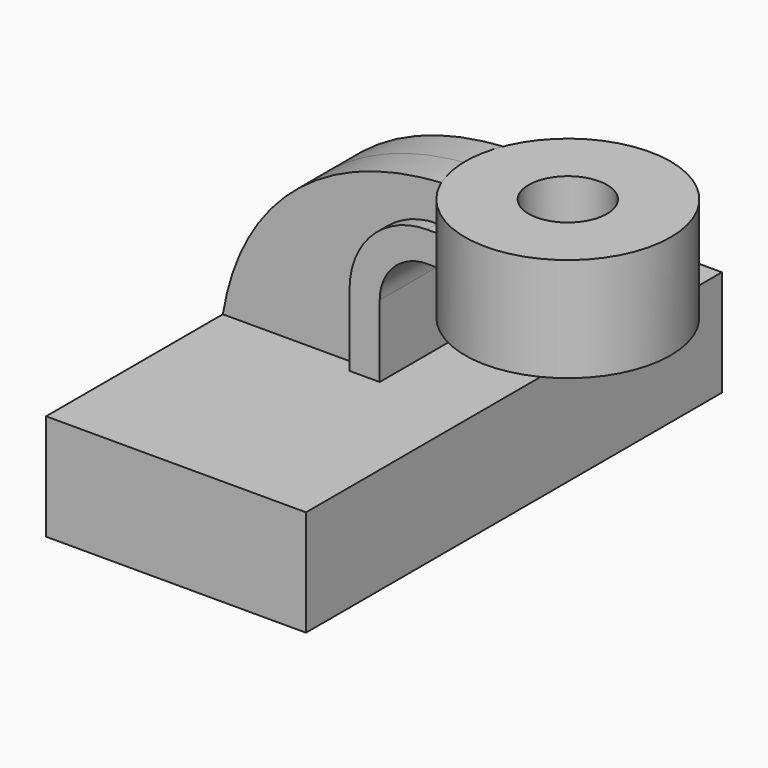
from build123d import *

# Parameters (mm, degrees)
F1_DEPTH = 63.5
F2_DEPTH = 9.525
F3_DEPTH = 12.7
F5_R     = 25.0978379379
F6_DEPTH = 25.4
F8_D     = 19.1516


with BuildPart() as f1:
    # F0 (on Front) → F1 (new body, symmetric)
    with BuildSketch(Plane.XZ):
        Polygon((-31.75, -12.9509741405), (31.75, -12.9509741405), (31.75, 12.9509741405), (9.1103371233, 12.9509741405), (1.7443363501, 12.9509741405), (-31.75, 12.9509741405), align=None)
    extrude(amount=F1_DEPTH, both=True)

    # F0 (on Front) → F2 (join, symmetric)
    with BuildSketch(Plane.XZ):
        with BuildLine():
            add(Edge.make_bspline(
                [(-31.75, 12.9509741405), (-27.0471625327, 41.6362041566), (-4.8953407756, 58.3005508379), (25.1726394472, 58.7224372514)],
                knots=[0, 0, 0, 0, 73.042547306, 73.042547306, 73.042547306, 73.042547306], degree=3))
            Line((-31.75, 12.9509741405), (1.7443363501, 12.9509741405))
            Line((1.7443363501, 12.9509741405), (1.7443363501, 30.5575896055))
            ThreePointArc((1.7443363501, 30.5575896055), (7.2928233486, 43.9528221678), (20.688055911, 49.5013091663))
            Line((20.688055911, 49.5013091663), (25.1726394472, 49.5013091663))
            Line((25.1726394472, 49.5013091663), (25.1726394472, 58.7224372514))
        make_face()
    extrude(amount=F2_DEPTH, both=True)

    # F0 (on Front) → F3 (join, symmetric)
    with BuildSketch(Plane.XZ):
        with BuildLine():
            Line((1.7443363501, 12.9509741405), (9.1103371233, 12.9509741405))
            Line((9.1103371233, 12.9509741405), (9.1103371233, 30.5575896055))
            ThreePointArc((9.1103371233, 30.5575896055), (12.5013724455, 38.7442730709), (20.688055911, 42.1353083932))
            Line((20.688055911, 42.1353083932), (25.1726394472, 42.1353083932))
            Line((25.1726394472, 42.1353083932), (25.1726394472, 49.5013091663))
            Line((25.1726394472, 49.5013091663), (20.688055911, 49.5013091663))
            ThreePointArc((20.688055911, 49.5013091663), (7.2928233486, 43.9528221678), (1.7443363501, 30.5575896055))
            Line((1.7443363501, 30.5575896055), (1.7443363501, 12.9509741405))
        make_face()
    extrude(amount=F3_DEPTH, both=True)


with BuildPart() as f4:
    # F0 (on Front) → F4 (revolve)
    with BuildSketch(Plane.XZ):
        Polygon((64.6507700858, 58.7224372514), (44.9117047665, 58.7224372514), (44.9117047665, 49.5013091663), (44.9117047665, 42.1353083932), (44.9117047665, 35.1127609611), (64.6507700858, 35.1127609611), align=None)
    revolve(axis=Axis((44.9117047665, 0, 46.9175991062), (0, 0, -1)))

    # F5 (on face) → F6 (join)
    with BuildSketch(Plane.XY.offset(58.7224372514)):
        with Locations((44.9117047665, 0)):
            Circle(F5_R)
    extrude(amount=-F6_DEPTH)

    # F8 (through all)
    with Locations(Plane.XY.offset(58.7224372514)):
        with Locations((44.9117047665, 0)):
            Hole(F8_D / 2)


solid = Compound([f1.part, f4.part])
